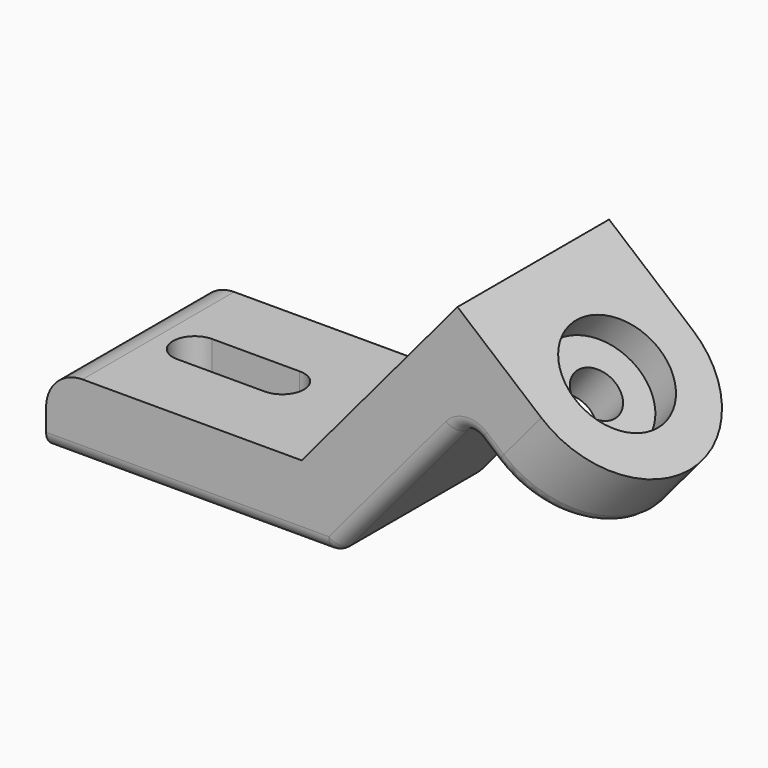
from build123d import *

# Parameters (mm, degrees)
F1_DEPTH    = 13
F2_T1_DEPTH = 75
F3_R        = 2
F4_R        = 7.3
F5_DEPTH    = 4.4
F6_R        = 3.3
F7_DEPTH    = 59.0732481421
F9_DEPTH    = 10.001
F10_R       = 5


# Not quite as in the source:
# - a fillet or chamfer that OpenCascade refuses, or shapes differently, is made with other operations: its cross-section is extruded or revolved along the edge and cut away or added


with BuildPart() as f1:
    # F0 (on Front) → F1 (new body, symmetric)
    with BuildSketch(Plane.XZ):
        Polygon((-38.8, 8), (-38.8, 0), (0, 0), (18.6408406809, 22.2152888505), (33.9617295433, 9.3595366567), (39.1040304208, 15.4878922017), (17.6547860135, 33.4859452729), (-3.7304612652, 8), align=None)
        Polygon((0, 0), (-38.8, 0), (-38.8, -2), (0.9326153163, -2), (18.8873543478, 19.3976247448), (32.6761543239, 7.8274477705), (33.9617295433, 9.3595366567), (18.6408406809, 22.2152888505), align=None)
    extrude(amount=F1_DEPTH, both=True)

    # F2: fillet of radius 13 on 2 edges, made by hand

    # F2_s2 → F2_t1 (cut)
    with BuildSketch(Plane(origin=(-3.5353318533, 0, -4.2132444372), x_dir=(0, 1, 0), z_dir=(0.6427876097, 0, 0.7660444431))):
        with BuildLine():
            ThreePointArc((0, -20), (-9.1923881554, -16.1923881554), (-13, -7))
            Line((-13, -7), (-13, -20))
            Line((-13, -20), (0, -20))
        make_face()
        with BuildLine():
            ThreePointArc((0, -20), (9.1923881554, -16.1923881554), (13, -7))
            Line((13, -7), (13, -20))
            Line((13, -20), (0, -20))
        make_face()
    extrude(amount=F2_T1_DEPTH, mode=Mode.SUBTRACT)

    # F3
    f3_edges = [f1.edges().sort_by_distance(p)[0] for p in [
        (18.887354, 0, 19.397625),
        (20.802465, -13, 17.790656),
        (29.759354, -9.192388, 10.274933),
        (29.759354, 9.192388, 10.274933),
        (20.802465, 13, 17.790656),
        (0.932615, 0, -2),
        (-18.933692, -13, -2),
        (-18.933692, 13, -2),
        (9.909985, 13, 8.698812),
        (9.909985, -13, 8.698812),
    ]]
    fillet(f3_edges, radius=F3_R)

    # F4 (on face) → F5 (cut)
    with BuildSketch(Plane(origin=(23.7831415584, 0, 28.3436443954), x_dir=(0.7660444431, 0, -0.6427876097), z_dir=(0.6427876097, 0, 0.7660444431))):
        with Locations((7, 0)):
            Circle(F4_R)
    extrude(amount=-F5_DEPTH, mode=Mode.SUBTRACT)

    # F6 (on face) → F7 (cut, through all)
    with BuildSketch(Plane(origin=(20.9548760758, 0, 24.9730488457), x_dir=(0.7660444431, 0, -0.6427876097), z_dir=(0.6427876097, 0, 0.7660444431))):
        with Locations((7, 0)):
            Circle(F6_R)
    extrude(amount=-F7_DEPTH, mode=Mode.SUBTRACT)

    # F8 (on face) → F9 (cut, through all)
    with BuildSketch(Plane.XY.offset(8)):
        with BuildLine():
            ThreePointArc((-28.8, 3), (-31.8, 0), (-28.8, -3))
            Line((-28.8, -3), (-16.8, -3))
            ThreePointArc((-16.8, -3), (-13.8, 0), (-16.8, 3))
            Line((-16.8, 3), (-28.8, 3))
        make_face()
    extrude(amount=-F9_DEPTH, mode=Mode.SUBTRACT)

    # F10
    f10_edges = [f1.edges().sort_by_distance(p)[0] for p in [
        (-38.8, 0, 8),
    ]]
    fillet(f10_edges, radius=F10_R)


solid = f1.part
